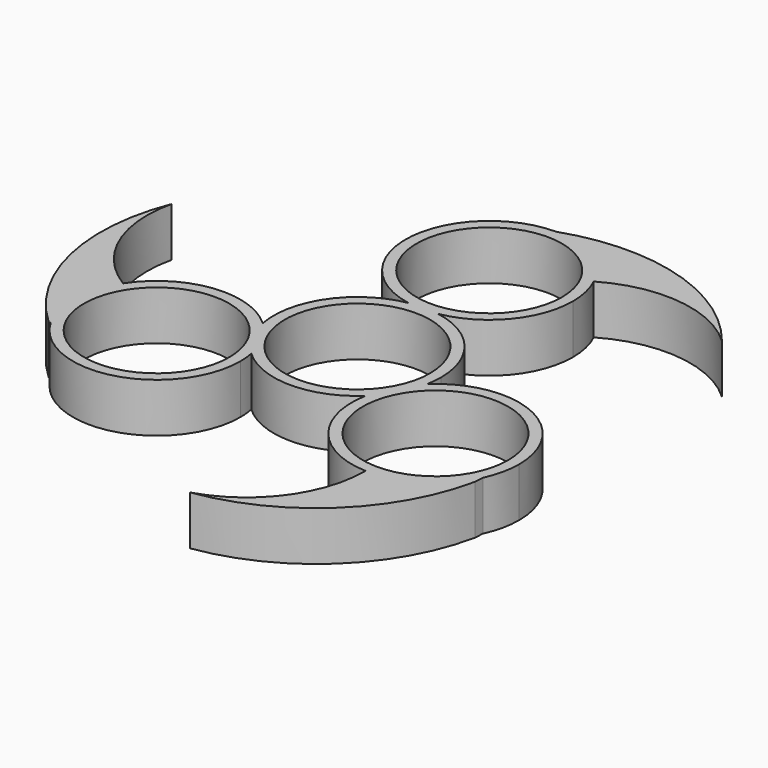
from build123d import *

# Parameters (mm, degrees)
F0_R     = 11.2522
F1_DEPTH = 7.62
F2_DEPTH = 5.334


with BuildPart() as f1:
    # F0 (on Top) → F1 (new body)
    with BuildSketch(Plane.XY):
        with BuildLine():
            ThreePointArc((12.7369944105, -2.4049880816), (12.9056707985, -1.2077481218), (12.962059801, 0))
            ThreePointArc((12.962059801, 0), (9.9385595014, 8.321059387), (2.2785680744, 12.7602163702))
            ThreePointArc((2.2785680744, 12.7602163702), (0, 12.5583729394), (-2.2785680744, 12.7602163702))
            ThreePointArc((-2.2785680744, 12.7602163702), (-10.6706436404, 7.3588286149), (-12.7369944105, -2.4049880816))
            ThreePointArc((-12.7369944105, -2.4049880816), (-10.231616704, -5.6270418202), (-8.8523481214, -9.4684173452))
            ThreePointArc((-8.8523481214, -9.4684173452), (0, -12.962059801), (8.8523481214, -9.4684173452))
            ThreePointArc((8.8523481214, -9.4684173452), (10.231616704, -5.6270418202), (12.7369944105, -2.4049880816))
        make_face()
        Circle(F0_R, mode=Mode.SUBTRACT)
        with BuildLine():
            ThreePointArc((-2.2785680744, 12.7602163702), (0, 12.5583729394), (2.2785680744, 12.7602163702))
            ThreePointArc((2.2785680744, 12.7602163702), (0, 12.962059801), (-2.2785680744, 12.7602163702))
        make_face()
        with BuildLine():
            ThreePointArc((-2.2785680744, 12.7602163702), (0, 12.962059801), (2.2785680744, 12.7602163702))
            ThreePointArc((2.2785680744, 12.7602163702), (9.9385595014, 17.1993733535), (12.962059801, 25.5204327404))
            ThreePointArc((12.962059801, 25.5204327404), (12.6382642104, 28.3995423305), (11.6830544332, 31.1348101232))
            ThreePointArc((11.6830544332, 31.1348101232), (6.9007644107, 36.492872981), (0, 38.4824925414))
            ThreePointArc((0, 38.4824925414), (-12.9115003379, 26.6641780399), (-2.2785680744, 12.7602163702))
        make_face()
        with Locations((0, 25.5204327404)):
            Circle(F0_R, mode=Mode.SUBTRACT)
        with BuildLine():
            ThreePointArc((34.5514023329, -11.8734054267), (26.7502692198, 0.0169196322), (12.7369944105, -2.4049880816))
            ThreePointArc((12.7369944105, -2.4049880816), (11.3577258278, -6.2463636065), (8.8523481214, -9.4684173452))
            ThreePointArc((8.8523481214, -9.4684173452), (11.4621329747, -19.9638084371), (21.1220092921, -24.8270378875))
            ThreePointArc((21.1220092921, -24.8270378875), (27.8669248008, -23.2139060833), (32.8148156049, -18.3544353272))
            ThreePointArc((32.8148156049, -18.3544353272), (33.0812954491, -17.869238349), (33.3268161418, -17.373106104))
            ThreePointArc((33.3268161418, -17.373106104), (34.2415524007, -14.6905990161), (34.5514023329, -11.8734054267))
        make_face()
        with Locations((21.5893425319, -11.8734054267)):
            Circle(F0_R, mode=Mode.SUBTRACT)
        with BuildLine():
            ThreePointArc((8.8523481214, -9.4684173452), (11.3577258278, -6.2463636065), (12.7369944105, -2.4049880816))
            ThreePointArc((12.7369944105, -2.4049880816), (10.231616704, -5.6270418202), (8.8523481214, -9.4684173452))
        make_face()
        with BuildLine():
            ThreePointArc((-8.8523481214, -9.4684173452), (-10.231616704, -5.6270418202), (-12.7369944105, -2.4049880816))
            ThreePointArc((-12.7369944105, -2.4049880816), (-11.3577258278, -6.2463636065), (-8.8523481214, -9.4684173452))
        make_face()
        with BuildLine():
            ThreePointArc((-8.8523481214, -9.4684173452), (-11.3577258278, -6.2463636065), (-12.7369944105, -2.4049880816))
            ThreePointArc((-12.7369944105, -2.4049880816), (-23.1489478225, 0.9944858388), (-32.4473199354, -4.7939053745))
            ThreePointArc((-32.4473199354, -4.7939053745), (-34.5466450824, -11.5222574559), (-32.8148156049, -18.3544353272))
            ThreePointArc((-32.8148156049, -18.3544353272), (-18.2345145916, -24.3937937504), (-8.6272827309, -11.8734054267))
            ThreePointArc((-8.6272827309, -11.8734054267), (-8.6836717334, -10.665657305), (-8.8523481214, -9.4684173452))
        make_face()
        with Locations((-21.5893425319, -11.8734054267)):
            Circle(F0_R, mode=Mode.SUBTRACT)
        with BuildLine():
            ThreePointArc((33.5095214822, 28.6722648172), (18.313797705, 38.902696715), (0, 38.4824925414))
            ThreePointArc((0, 38.4824925414), (6.9007644107, 36.492872981), (11.6830544332, 31.1348101232))
            ThreePointArc((11.6830544332, 31.1348101232), (23.0045235804, 33.5218836362), (33.5095214822, 28.6722648172))
        make_face()
        with BuildLine():
            ThreePointArc((32.8148156049, -18.3544353272), (27.8669248008, -23.2139060833), (21.1220092921, -24.8270378875))
            ThreePointArc((21.1220092921, -24.8270378875), (17.5285410214, -35.8252545336), (8.0761489747, -42.4980401738))
            ThreePointArc((8.0761489747, -42.4980401738), (24.3755164942, -34.6034732765), (33.2400792742, -18.8106554549))
            ThreePointArc((33.2400792742, -18.8106554549), (33.0293167827, -18.5808028908), (32.8148156049, -18.3544353272))
        make_face()
        with BuildLine():
            Line((33.2400792742, -18.8106554549), (33.3268161418, -17.373106104))
            ThreePointArc((33.3268161418, -17.373106104), (33.0812954491, -17.869238349), (32.8148156049, -18.3544353272))
            ThreePointArc((32.8148156049, -18.3544353272), (33.0293167827, -18.5808028908), (33.2400792742, -18.8106554549))
        make_face()
        with BuildLine():
            ThreePointArc((-32.8148156049, -18.3544353272), (-34.5466450824, -11.5222574559), (-32.4473199354, -4.7939053745))
            ThreePointArc((-32.4473199354, -4.7939053745), (-39.8779765619, 3.7961234456), (-40.8424568889, 15.1130590171))
            ThreePointArc((-40.8424568889, 15.1130590171), (-42.2015912045, -2.7503305518), (-33.2137545387, -18.2476440302))
            ThreePointArc((-33.2137545387, -18.2476440302), (-33.0145748071, -18.3021220393), (-32.8148156049, -18.3544353272))
        make_face()
    extrude(amount=F1_DEPTH)

    # F0 (on Top) → F2 (join)
    with BuildSketch(Plane.XY):
        with BuildLine():
            ThreePointArc((32.8148156049, -18.3544353272), (27.8669248008, -23.2139060833), (21.1220092921, -24.8270378875))
            ThreePointArc((21.1220092921, -24.8270378875), (17.5285410214, -35.8252545336), (8.0761489747, -42.4980401738))
            ThreePointArc((8.0761489747, -42.4980401738), (24.3755164942, -34.6034732765), (33.2400792742, -18.8106554549))
            ThreePointArc((33.2400792742, -18.8106554549), (33.0293167827, -18.5808028908), (32.8148156049, -18.3544353272))
        make_face()
        with BuildLine():
            ThreePointArc((-32.8148156049, -18.3544353272), (-34.5466450824, -11.5222574559), (-32.4473199354, -4.7939053745))
            ThreePointArc((-32.4473199354, -4.7939053745), (-39.8779765619, 3.7961234456), (-40.8424568889, 15.1130590171))
            ThreePointArc((-40.8424568889, 15.1130590171), (-42.2015912045, -2.7503305518), (-33.2137545387, -18.2476440302))
            ThreePointArc((-33.2137545387, -18.2476440302), (-33.0145748071, -18.3021220393), (-32.8148156049, -18.3544353272))
        make_face()
        with BuildLine():
            ThreePointArc((33.5095214822, 28.6722648172), (18.313797705, 38.902696715), (0, 38.4824925414))
            ThreePointArc((0, 38.4824925414), (6.9007644107, 36.492872981), (11.6830544332, 31.1348101232))
            ThreePointArc((11.6830544332, 31.1348101232), (23.0045235804, 33.5218836362), (33.5095214822, 28.6722648172))
        make_face()
        with BuildLine():
            ThreePointArc((-2.2785680744, 12.7602163702), (0, 12.962059801), (2.2785680744, 12.7602163702))
            ThreePointArc((2.2785680744, 12.7602163702), (9.9385595014, 17.1993733535), (12.962059801, 25.5204327404))
            ThreePointArc((12.962059801, 25.5204327404), (12.6382642104, 28.3995423305), (11.6830544332, 31.1348101232))
            ThreePointArc((11.6830544332, 31.1348101232), (6.9007644107, 36.492872981), (0, 38.4824925414))
            ThreePointArc((0, 38.4824925414), (-12.9115003379, 26.6641780399), (-2.2785680744, 12.7602163702))
        make_face()
        with Locations((0, 25.5204327404)):
            Circle(F0_R, mode=Mode.SUBTRACT)
        with BuildLine():
            ThreePointArc((12.7369944105, -2.4049880816), (12.9056707985, -1.2077481218), (12.962059801, 0))
            ThreePointArc((12.962059801, 0), (9.9385595014, 8.321059387), (2.2785680744, 12.7602163702))
            ThreePointArc((2.2785680744, 12.7602163702), (0, 12.5583729394), (-2.2785680744, 12.7602163702))
            ThreePointArc((-2.2785680744, 12.7602163702), (-10.6706436404, 7.3588286149), (-12.7369944105, -2.4049880816))
            ThreePointArc((-12.7369944105, -2.4049880816), (-10.231616704, -5.6270418202), (-8.8523481214, -9.4684173452))
            ThreePointArc((-8.8523481214, -9.4684173452), (0, -12.962059801), (8.8523481214, -9.4684173452))
            ThreePointArc((8.8523481214, -9.4684173452), (10.231616704, -5.6270418202), (12.7369944105, -2.4049880816))
        make_face()
        Circle(F0_R, mode=Mode.SUBTRACT)
        with BuildLine():
            ThreePointArc((34.5514023329, -11.8734054267), (26.7502692198, 0.0169196322), (12.7369944105, -2.4049880816))
            ThreePointArc((12.7369944105, -2.4049880816), (11.3577258278, -6.2463636065), (8.8523481214, -9.4684173452))
            ThreePointArc((8.8523481214, -9.4684173452), (11.4621329747, -19.9638084371), (21.1220092921, -24.8270378875))
            ThreePointArc((21.1220092921, -24.8270378875), (27.8669248008, -23.2139060833), (32.8148156049, -18.3544353272))
            ThreePointArc((32.8148156049, -18.3544353272), (33.0812954491, -17.869238349), (33.3268161418, -17.373106104))
            ThreePointArc((33.3268161418, -17.373106104), (34.2415524007, -14.6905990161), (34.5514023329, -11.8734054267))
        make_face()
        with Locations((21.5893425319, -11.8734054267)):
            Circle(F0_R, mode=Mode.SUBTRACT)
        with BuildLine():
            ThreePointArc((8.8523481214, -9.4684173452), (11.3577258278, -6.2463636065), (12.7369944105, -2.4049880816))
            ThreePointArc((12.7369944105, -2.4049880816), (10.231616704, -5.6270418202), (8.8523481214, -9.4684173452))
        make_face()
        with BuildLine():
            ThreePointArc((-2.2785680744, 12.7602163702), (0, 12.5583729394), (2.2785680744, 12.7602163702))
            ThreePointArc((2.2785680744, 12.7602163702), (0, 12.962059801), (-2.2785680744, 12.7602163702))
        make_face()
        with BuildLine():
            ThreePointArc((-8.8523481214, -9.4684173452), (-10.231616704, -5.6270418202), (-12.7369944105, -2.4049880816))
            ThreePointArc((-12.7369944105, -2.4049880816), (-11.3577258278, -6.2463636065), (-8.8523481214, -9.4684173452))
        make_face()
        with BuildLine():
            ThreePointArc((-8.8523481214, -9.4684173452), (-11.3577258278, -6.2463636065), (-12.7369944105, -2.4049880816))
            ThreePointArc((-12.7369944105, -2.4049880816), (-23.1489478225, 0.9944858388), (-32.4473199354, -4.7939053745))
            ThreePointArc((-32.4473199354, -4.7939053745), (-34.5466450824, -11.5222574559), (-32.8148156049, -18.3544353272))
            ThreePointArc((-32.8148156049, -18.3544353272), (-18.2345145916, -24.3937937504), (-8.6272827309, -11.8734054267))
            ThreePointArc((-8.6272827309, -11.8734054267), (-8.6836717334, -10.665657305), (-8.8523481214, -9.4684173452))
        make_face()
        with Locations((-21.5893425319, -11.8734054267)):
            Circle(F0_R, mode=Mode.SUBTRACT)
    extrude(amount=F2_DEPTH)


solid = f1.part
